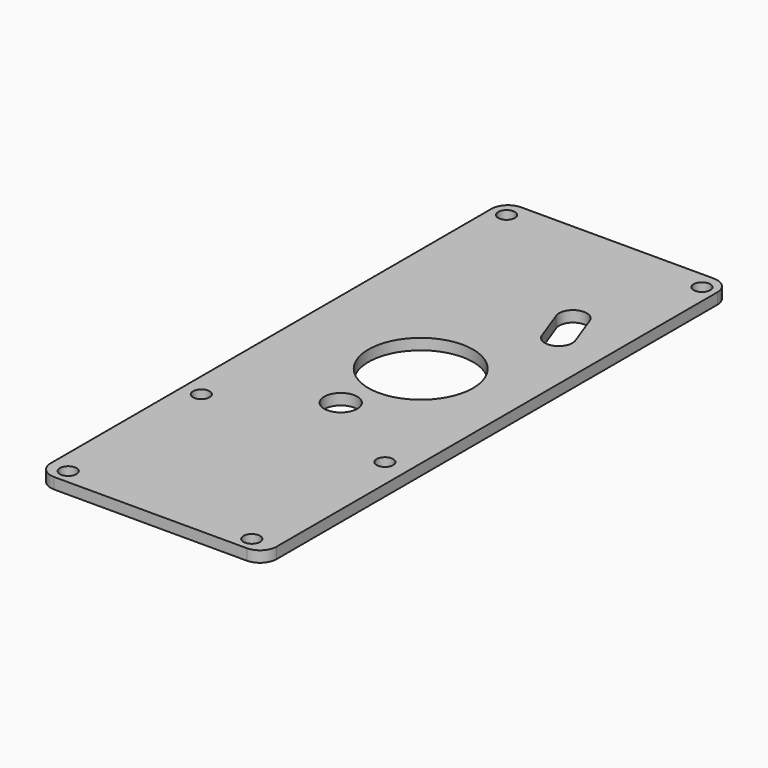
from build123d import *

# Parameters (mm, degrees)
F0_W     = 41
F0_H     = 106
F0_R     = 1.5
F0_R_2   = 5.05
F0_R_3   = 2
F0_R_4   = 3
F0_R_5   = 9.5
F1_DEPTH = 2
F2_R     = 3


# Not quite as in the source:
# - a feature names something its author has since deleted; it is built from what else it names


with BuildPart() as f1:
    # F0 (on Top) → F1 (new body)
    with BuildSketch(Plane.XY):
        with Locations((-1.1801278293, -1.1353523731)):
            Rectangle(F0_W, F0_H)
        with Locations((-18.2301278293, -51.4703523731)):
            Circle(F0_R, mode=Mode.SUBTRACT)
        with Locations((-6.776117335, -33.481924504)):
            Circle(F0_R_2, mode=Mode.SUBTRACT)
        with Locations((-18.2301278293, -21.2703523731)):
            Circle(F0_R, mode=Mode.SUBTRACT)
        with Locations((-11.8353097141, -18.4490393624)):
            Circle(F0_R_3, mode=Mode.SUBTRACT)
        with BuildLine():
            ThreePointArc((0.9913514778, -28.481924504), (-4.9415118708, -25.855220261), (-8.0481067447, -20.1589485871))
            Line((-8.0481067447, -20.1589485871), (9.9913514778, -20.516399593))
            Line((9.9913514778, -20.516399593), (9.9913514778, -46.516399593))
            Line((9.9913514778, -46.516399593), (-8.0481067447, -46.804900421))
            ThreePointArc((-8.0481067447, -46.804900421), (-4.9415118708, -41.1086287471), (0.9913514778, -38.481924504))
            Line((0.9913514778, -38.481924504), (0.9913514778, -28.481924504))
        make_face(mode=Mode.SUBTRACT)
        with Locations((15.0892422113, -51.4703523731)):
            Circle(F0_R, mode=Mode.SUBTRACT)
        with Locations((-1.1801278293, -10.9442314133)):
            Circle(F0_R_4, mode=Mode.SUBTRACT)
        with Locations((15.0892422113, -21.2703523731)):
            Circle(F0_R, mode=Mode.SUBTRACT)
        with Locations((-11.8353097141, -0.1353523731)):
            Circle(F0_R_3, mode=Mode.SUBTRACT)
        with Locations((-11.8353097141, 18.1783346161)):
            Circle(F0_R_3, mode=Mode.SUBTRACT)
        with Locations((-18.8301271707, 48.7366476269)):
            Circle(F0_R, mode=Mode.SUBTRACT)
        with Locations((-6.776117335, 33.2112197578)):
            Circle(F0_R_2, mode=Mode.SUBTRACT)
        with Locations((1.1698721707, 4.2646476269)):
            Circle(F0_R_5, mode=Mode.SUBTRACT)
        with BuildLine():
            ThreePointArc((0.9913514778, 38.2112197578), (-4.9415118708, 40.8379240009), (-8.0481067447, 46.5341956747))
            Line((-8.0481067447, 46.5341956747), (9.9913514778, 46.2456948468))
            Line((9.9913514778, 46.2456948468), (9.9913514778, 31.7237218389))
            ThreePointArc((9.9913514778, 31.7237218389), (10.4081379557, 31.2391097076), (10.6884153726, 30.6646495649))
            Line((10.6884153726, 30.6646495649), (12.8669505005, 24.7255908967))
            ThreePointArc((12.8669505005, 24.7255908967), (12.9813448828, 24.3018570593), (13.0198721707, 23.8646476269))
            ThreePointArc((13.0198721707, 23.8646476269), (12.0896967258, 21.9189727141), (9.9913514778, 21.4211530234))
            Line((9.9913514778, 21.4211530234), (9.9913514778, 20.2456948468))
            Line((9.9913514778, 20.2456948468), (-8.0481067447, 19.8882438409))
            ThreePointArc((-8.0481067447, 19.8882438409), (-4.9415118708, 25.5845155147), (0.9913514778, 28.2112197578))
            Line((0.9913514778, 28.2112197578), (0.9913514778, 38.2112197578))
        make_face(mode=Mode.SUBTRACT)
        with Locations((16.6392421771, 48.7366476269)):
            Circle(F0_R, mode=Mode.SUBTRACT)
        with BuildLine():
            Line((9.9913514778, -20.516399593), (-8.0481067447, -20.1589485871))
            ThreePointArc((-8.0481067447, -20.1589485871), (-4.9415118708, -25.855220261), (0.9913514778, -28.481924504))
            Line((0.9913514778, -28.481924504), (0.9913514778, -38.481924504))
            ThreePointArc((0.9913514778, -38.481924504), (-4.9415118708, -41.1086287471), (-8.0481067447, -46.804900421))
            Line((-8.0481067447, -46.804900421), (9.9913514778, -46.516399593))
            Line((9.9913514778, -46.516399593), (9.9913514778, -20.516399593))
        make_face()
        with Locations((-2.2937730764, -41.981924504)):
            Circle(F0_R, mode=Mode.SUBTRACT)
        with Locations((-2.2937730764, -24.981924504)):
            Circle(F0_R, mode=Mode.SUBTRACT)
        with BuildLine():
            Line((9.9913514778, 46.2456948468), (-8.0481067447, 46.5341956747))
            ThreePointArc((-8.0481067447, 46.5341956747), (-4.9415118708, 40.8379240009), (0.9913514778, 38.2112197578))
            Line((0.9913514778, 38.2112197578), (0.9913514778, 28.2112197578))
            ThreePointArc((0.9913514778, 28.2112197578), (-4.9415118708, 25.5845155147), (-8.0481067447, 19.8882438409))
            Line((-8.0481067447, 19.8882438409), (9.9913514778, 20.2456948468))
            Line((9.9913514778, 20.2456948468), (9.9913514778, 21.4211530234))
            ThreePointArc((9.9913514778, 21.4211530234), (8.9707387909, 21.9024586015), (8.2657292668, 22.7835186943))
            ThreePointArc((8.2657292668, 22.7835186943), (8.1741724057, 22.9999554201), (8.1033430916, 23.2240329142))
            Line((8.1033430916, 23.2240329142), (5.9741724057, 28.9999554201))
            ThreePointArc((5.9741724057, 28.9999554201), (6.9168863609, 31.9338578186), (9.9913514778, 31.7237218389))
            Line((9.9913514778, 31.7237218389), (9.9913514778, 46.2456948468))
        make_face()
        with Locations((-2.2937730764, 24.7112197578)):
            Circle(F0_R, mode=Mode.SUBTRACT)
        with Locations((-2.2937730764, 41.7112197578)):
            Circle(F0_R, mode=Mode.SUBTRACT)
        with Locations((-6.776117335, 33.2112197578)):
            Circle(F0_R_2)
        with Locations((-6.776117335, -33.481924504)):
            Circle(F0_R_2)
        with Locations((-11.8353097141, -18.4490393624)):
            Circle(F0_R_3)
        with Locations((-11.8353097141, -0.1353523731)):
            Circle(F0_R_3)
        with Locations((-11.8353097141, 18.1783346161)):
            Circle(F0_R_3)
        with Locations((-2.2937730764, -24.981924504)):
            Circle(F0_R)
        with Locations((-2.2937730764, -41.981924504)):
            Circle(F0_R)
        with Locations((-2.2937730764, 24.7112197578)):
            Circle(F0_R)
        with Locations((-2.2937730764, 41.7112197578)):
            Circle(F0_R)
    extrude(amount=F1_DEPTH)

    # F2
    f2_edges = [f1.edges().sort_by_distance(p)[0] for p in [
        (-21.680128, 51.864648, 1),
        (-21.680128, -54.135352, 1),
        (19.319872, -54.135352, 1),
        (19.319872, 51.864648, 1),
    ]]
    fillet(f2_edges, radius=F2_R)


solid = f1.part
